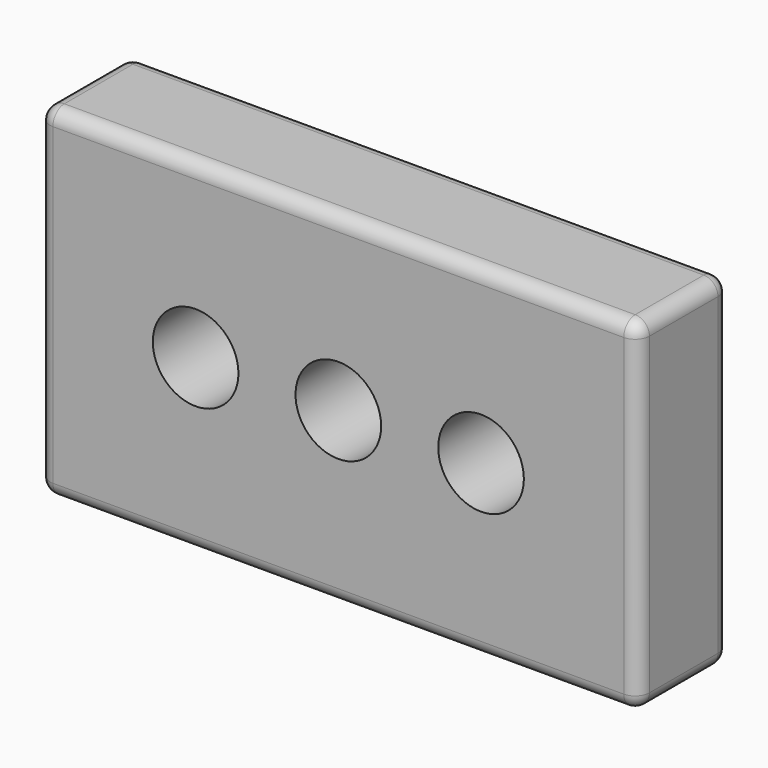
from build123d import *

# Parameters (mm, degrees)
F0_W         = 266.7
F0_H         = 152.4
F0_R         = 19.05
F1_DEPTH     = 50.8
F2_R         = 6.35
F3_R         = 6.35
F4_R         = 6.35
F5_R         = 6.35
F6_T1_DEPTH  = 38.1
F6_S5_W      = 6.35
F6_S5_H      = 6.35
F6_T6_DEPTH  = 6.35
F6_S11_W     = 6.35
F6_S11_H     = 6.35
F6_T12_DEPTH = 6.35


# Not quite as in the source:
# - a fillet or chamfer that OpenCascade refuses, or shapes differently, is made with other operations: its cross-section is extruded or revolved along the edge and cut away or added


with BuildPart() as f1:
    # F0 (on Front) → F1 (new body)
    with BuildSketch(Plane.XZ):
        Rectangle(F0_W, F0_H)
        with Locations((-63.5, 0)):
            Circle(F0_R, mode=Mode.SUBTRACT)
        Circle(F0_R, mode=Mode.SUBTRACT)
        with Locations((63.5, 0)):
            Circle(F0_R, mode=Mode.SUBTRACT)
    extrude(amount=F1_DEPTH)

    # F2
    f2_edges = [f1.edges().sort_by_distance(p)[0] for p in [
        (0, -50.8, 76.2),
    ]]
    fillet(f2_edges, radius=F2_R)

    # F3
    f3_edges = [f1.edges().sort_by_distance(p)[0] for p in [
        (133.35, -50.8, -3.175),
    ]]
    fillet(f3_edges, radius=F3_R)

    # F4
    f4_edges = [f1.edges().sort_by_distance(p)[0] for p in [
        (-3.175, -50.8, -76.2),
        (-133.35, -50.8, -3.175),
    ]]
    fillet(f4_edges, radius=F4_R)

    # F5
    f5_edges = [f1.edges().sort_by_distance(p)[0] for p in [
        (0, 0, 76.2),
    ]]
    fillet(f5_edges, radius=F5_R)

    # F6: fillet of radius 6.35 on 1 edges, made by hand

    # F6_s2 → F6_t1 (cut)
    with BuildSketch(Plane.XZ.offset(6.35)):
        with BuildLine():
            ThreePointArc((-127, -76.2), (-131.4901280605, -74.3401280605), (-133.35, -69.85))
            Line((-133.35, -69.85), (-133.35, -76.2))
            Line((-133.35, -76.2), (-127, -76.2))
        make_face()
    extrude(amount=F6_T1_DEPTH, mode=Mode.SUBTRACT)


with BuildPart() as f6_tool4:
    # F6_s5 → F6_t6 (new body)
    with BuildSketch(Plane.XY.offset(-69.85)):
        with Locations((-130.175, -3.175)):
            Rectangle(F6_S5_W, F6_S5_H)
    extrude(amount=-F6_T6_DEPTH)

    # F6_s7 → F6_t8 (revolve, cut)
    with BuildSketch(Plane(origin=(-127, -6.35, -69.85), x_dir=(0.7071067812, -0.7071067812, 0), z_dir=(0.7071067812, 0.7071067812, 0))):
        with BuildLine():
            ThreePointArc((0, -6.35), (6.35, 0), (0, 6.35))
            Line((0, 6.35), (0, -6.35))
        make_face()
    revolve(axis=Axis((-127, -6.35, -69.85), (0, 0, -1)), mode=Mode.SUBTRACT)


with BuildPart() as f1_1:
    add(f1.part)

    # F6_t3: cut F6_tool4
    add(f6_tool4.part, mode=Mode.SUBTRACT)


with BuildPart() as f6_tool10:
    # F6_s11 → F6_t12 (new body)
    with BuildSketch(Plane.XY.offset(-69.85)):
        with Locations((-130.175, -47.625)):
            Rectangle(F6_S11_W, F6_S11_H)
    extrude(amount=-F6_T12_DEPTH)

    # F6_s13 → F6_t14 (revolve, cut)
    with BuildSketch(Plane(origin=(-127, -44.45, -69.85), x_dir=(0.7071067812, 0.7071067812, 0), z_dir=(-0.7071067812, 0.7071067812, 0))):
        with BuildLine():
            ThreePointArc((0, -6.35), (6.35, 0), (0, 6.35))
            Line((0, 6.35), (0, -6.35))
        make_face()
    revolve(axis=Axis((-127, -44.45, -69.85), (0, 0, -1)), mode=Mode.SUBTRACT)


with BuildPart() as f1_2:
    add(f1_1.part)

    # F6_t9: cut F6_tool10
    add(f6_tool10.part, mode=Mode.SUBTRACT)


solid = f1_2.part
